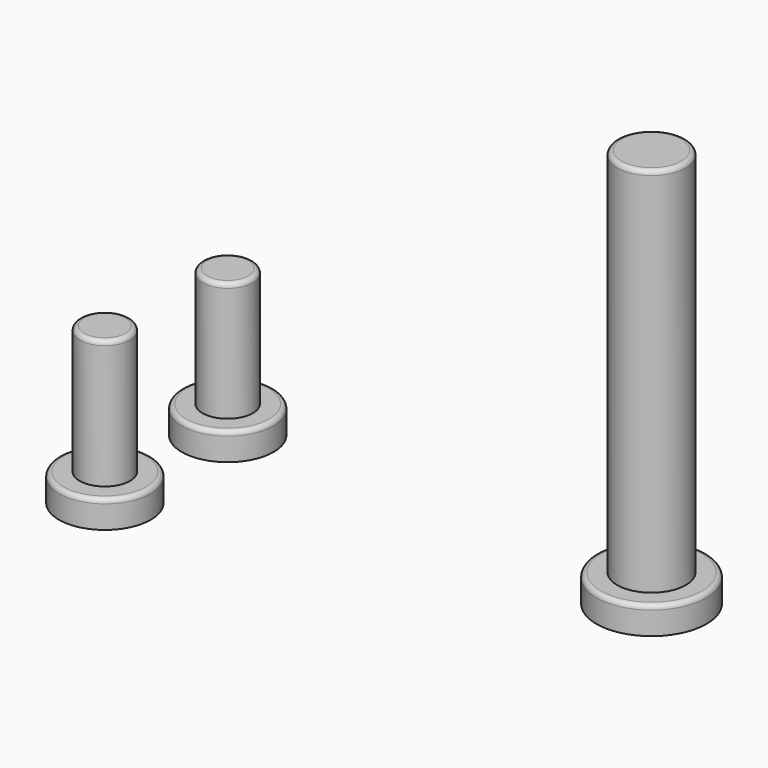
from build123d import *

# Parameters (mm, degrees)
F0_R          = 1.375
F1_DEPTH      = 7
F0_R_2        = 2.5
F2_DEPTH      = 1.5
F4_R          = 1.375
F5_DEPTH      = 6.5
F4_R_2        = 2.5
F6_DEPTH      = 1.5
F8_R          = 1.875
F9_DEPTH      = 20.25
F8_R_2        = 3
F10_DEPTH     = 1.5
F11_TEXT_SIZE = 6.5606484573
F7_TEXT_SIZE  = 5.1624333291
F3_TEXT_SIZE  = 5.4223556407
F12_DEPTH     = 0.25
F13_R         = 0.25
F13_2_R       = 0.25
F13_3_R       = 0.25


# Not quite as in the source:
# - Text() gives the source's letters only with a copy of the font that has no kerning and outlines rounded to 1/6400 em; it was checked with that copy


with BuildPart() as f1:
    # F0 (on Top) → F1 (new body)
    with BuildSketch(Plane.XY):
        with Locations((-13.665756549, -9.0186396553)):
            Circle(F0_R)
    extrude(amount=F1_DEPTH)

    # F0 (on Top) → F2 (join)
    with BuildSketch(Plane.XY):
        with Locations((-13.665756549, -9.0186396553)):
            Circle(F0_R_2)
        with Locations((-13.665756549, -9.0186396553)):
            Circle(F0_R, mode=Mode.SUBTRACT)
        with Locations((-13.665756549, -9.0186396553)):
            Circle(F0_R)
    extrude(amount=-F2_DEPTH)


with BuildPart() as f5:
    # F4 (on Top) → F5 (new body)
    with BuildSketch(Plane.XY):
        with Locations((-13.485272433, -0.8791188925)):
            Circle(F4_R)
    extrude(amount=F5_DEPTH)

    # F4 (on Top) → F6 (join)
    with BuildSketch(Plane.XY):
        with Locations((-13.485272433, -0.8791188925)):
            Circle(F4_R_2)
        with Locations((-13.485272433, -0.8791188925)):
            Circle(F4_R, mode=Mode.SUBTRACT)
        with Locations((-13.485272433, -0.8791188925)):
            Circle(F4_R)
    extrude(amount=-F6_DEPTH)


with BuildPart() as f9:
    # F8 (on Top) → F9 (new body)
    with BuildSketch(Plane.XY):
        with Locations((10.2923819795, -1.7406290863)):
            Circle(F8_R)
    extrude(amount=F9_DEPTH)

    # F8 (on Top) → F10 (join)
    with BuildSketch(Plane.XY):
        with Locations((10.2923819795, -1.7406290863)):
            Circle(F8_R_2)
        with Locations((10.2923819795, -1.7406290863)):
            Circle(F8_R, mode=Mode.SUBTRACT)
        with Locations((10.2923819795, -1.7406290863)):
            Circle(F8_R)
    extrude(amount=-F10_DEPTH)


with BuildPart() as f12_tool:
    # F11 (on face) + F7 (on face) + F3 (on face) → F12 (new body)
    with BuildSketch(Plane(origin=(0, 0, -1.5), x_dir=(1, 0, 0), z_dir=(0, 0, -1))):
        with Locations((8.442586645, -0.6212043584)):
            Text('F', F11_TEXT_SIZE, font='Open Sans', font_style=FontStyle.BOLD, text_align=(TextAlign.LEFT, TextAlign.BOTTOM))
    with BuildSketch(Plane(origin=(0, 0, -1.5), x_dir=(1, 0, 0), z_dir=(0, 0, -1))):
        with Locations((-15.1574168535, -0.979357106)):
            Text('P', F7_TEXT_SIZE, font='Open Sans', font_style=FontStyle.BOLD, text_align=(TextAlign.LEFT, TextAlign.BOTTOM))
    with BuildSketch(Plane(origin=(0, 0, -1.5), x_dir=(1, 0, 0), z_dir=(0, 0, -1))):
        with Locations((-15.2276491464, 7.0665916247)):
            Text('S', F3_TEXT_SIZE, font='Open Sans', font_style=FontStyle.BOLD, text_align=(TextAlign.LEFT, TextAlign.BOTTOM))
    extrude(amount=-F12_DEPTH)


with BuildPart() as f1_1:
    add(f1.part)

    # F12: cut by f12_tool
    add(f12_tool.part, mode=Mode.SUBTRACT)

    # F13
    f13_edges = [f1_1.edges().sort_by_distance(p)[0] for p in [
        (-16.165757, -9.01864, 0),
        (-15.040757, -9.01864, 7),
    ]]
    fillet(f13_edges, radius=F13_R)


with BuildPart() as f5_1:
    add(f5.part)

    # F12: cut by f12_tool
    add(f12_tool.part, mode=Mode.SUBTRACT)

    # F13#2
    f13_2_edges = [f5_1.edges().sort_by_distance(p)[0] for p in [
        (-15.985272, -0.879119, 0),
        (-14.860272, -0.879119, 6.5),
    ]]
    fillet(f13_2_edges, radius=F13_2_R)


with BuildPart() as f9_1:
    add(f9.part)

    # F12: cut by f12_tool
    add(f12_tool.part, mode=Mode.SUBTRACT)

    # F13#3
    f13_3_edges = [f9_1.edges().sort_by_distance(p)[0] for p in [
        (7.292382, -1.740629, 0),
        (8.417382, -1.740629, 20.25),
    ]]
    fillet(f13_3_edges, radius=F13_3_R)


solid = Compound([f1_1.part, f5_1.part, f9_1.part])
